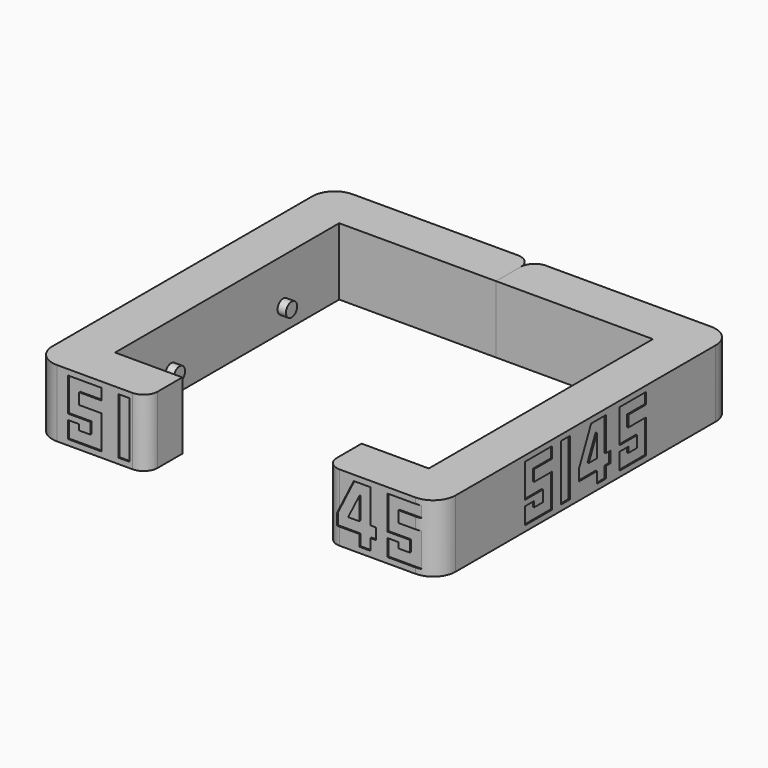
from build123d import *

# Parameters (mm, degrees)
F1_DEPTH       = 15.24
F2_R           = 1.5875
F3_DEPTH       = 1.905
F5_DEPTH       = 15.24
F6_R           = 1.5875
F7_DEPTH       = 1.905
F8_W           = 2.54
F8_H           = 12.7
F9_DEPTH       = 0.79375
F11_DEPTH      = 0.79375
F12_W          = 2.54
F12_H          = 12.7
F13_DEPTH      = 0.79375
F14_W          = 2.54
F14_H          = 12.7
F15_DEPTH      = 0.79375
F16_W          = 2.54
F16_H          = 12.7
F17_DEPTH      = 0.79375
F19_DEPTH      = 0.79375
F20_R          = 5.08
F21_T1_DEPTH   = 40.64
F22_T1_DEPTH   = 31.115
F22_2_T1_DEPTH = 31.115
F23_DEPTH      = 0.5
F24_DEPTH      = 0.5
F25_DEPTH      = 0.5
F26_DEPTH      = 0.5
F27_DEPTH      = 0.5
F28_DEPTH      = 0.5


# Not quite as in the source:
# - a fillet or chamfer that OpenCascade refuses, or shapes differently, is made with other operations: its cross-section is extruded or revolved along the edge and cut away or added


with BuildPart() as f1:
    # F0 (on Top) → F1 (new body)
    with BuildSketch(Plane.XY):
        Polygon((0, 38.8312135783), (0, 28.6712135783), (35.56, 28.6712135783), (35.56, -34.8287864217), (20.32, -34.8287864217), (20.32, -44.9887864217), (45.72, -44.9887864217), (45.72, 38.8312135783), align=None)
    extrude(amount=F1_DEPTH)

    # F2 (on face) → F3 (join)
    with BuildSketch(Plane(origin=(35.56, 0, 0), x_dir=(0, -1, 0), z_dir=(-1, 0, 0))):
        with Locations((-12.7962135783, 5.08)):
            Circle(F2_R)
        with Locations((18.9537864217, 5.08)):
            Circle(F2_R)
    extrude(amount=F3_DEPTH)

    # F8 (on face) → F9 (cut)
    with BuildSketch(Plane.YZ.offset(45.72)):
        Polygon((-12.6037864217, 11.43), (-12.6037864217, 13.97), (-20.2237864217, 13.97), (-20.2237864217, 6.35), (-15.1437864217, 6.35), (-15.1437864217, 3.81), (-17.6837864217, 3.81), (-17.6837864217, 5.08), (-20.2237864217, 5.08), (-20.2237864217, 1.27), (-12.6037864217, 1.27), (-12.6037864217, 8.89), (-17.6837864217, 8.89), (-17.6837864217, 11.43), align=None)
        with Locations((-8.7937864217, 7.62)):
            Rectangle(F8_W, F8_H)
        Polygon((2.6362135783, 13.97), (-1.5439947518, 13.97), (-4.9837864217, 6.35), (-4.9837864217, 3.81), (0.0962135783, 3.81), (0.0962135783, 1.27), (2.6362135783, 1.27), (2.6362135783, 3.81), (3.9062135783, 3.81), (3.9062135783, 6.35), (2.6362135783, 6.35), align=None)
        Polygon((0.0962135783, 11.43), (0.0962135783, 6.35), (-2.1969808683, 6.35), align=None, mode=Mode.SUBTRACT)
        Polygon((14.0662135783, 11.43), (14.0662135783, 13.97), (6.4462135783, 13.97), (6.4462135783, 6.35), (11.5262135783, 6.35), (11.5262135783, 3.81), (8.9862135783, 3.81), (8.9862135783, 5.08), (6.4462135783, 5.08), (6.4462135783, 1.27), (14.0662135783, 1.27), (14.0662135783, 8.89), (8.9862135783, 8.89), (8.9862135783, 11.43), align=None)
    extrude(amount=-F9_DEPTH, mode=Mode.SUBTRACT)

    # F10 (on face) → F11 (cut)
    with BuildSketch(Plane.XZ.offset(44.9887864217)):
        Polygon((26.67, 13.97), (22.86, 6.35), (22.86, 3.81), (27.94, 3.81), (27.94, 1.27), (30.48, 1.27), (30.48, 3.81), (31.75, 3.81), (31.75, 6.35), (30.48, 6.35), (30.48, 13.97), align=None)
        Polygon((27.94, 11.43), (27.94, 6.35), (25.4, 6.35), align=None, mode=Mode.SUBTRACT)
        Polygon((41.91, 11.43), (41.91, 13.97), (34.29, 13.97), (34.29, 6.35), (39.37, 6.35), (39.37, 3.81), (36.83, 3.81), (36.83, 5.08), (34.29, 5.08), (34.29, 1.27), (41.91, 1.27), (41.91, 8.89), (36.83, 8.89), (36.83, 11.43), align=None)
    extrude(amount=-F11_DEPTH, mode=Mode.SUBTRACT)

    # F16 (on face) → F17 (cut)
    with BuildSketch(Plane(origin=(0, 38.8312135783, 0), x_dir=(-1, 0, 0), z_dir=(0, 1, 0))):
        Polygon((-8.89, 11.43), (-8.89, 13.97), (-16.51, 13.97), (-16.51, 6.35), (-11.43, 6.35), (-11.43, 3.81), (-13.97, 3.81), (-13.97, 5.08), (-16.51, 5.08), (-16.51, 1.27), (-8.89, 1.27), (-8.89, 8.89), (-13.97, 8.89), (-13.97, 11.43), align=None)
        with Locations((-5.08, 7.62)):
            Rectangle(F16_W, F16_H)
    extrude(amount=-F17_DEPTH, mode=Mode.SUBTRACT)

    # F21: fillet of radius 5.08 on 2 edges, made by hand

    # F21_s2 → F21_t1 (cut)
    with BuildSketch(Plane.XY.offset(-12.7)):
        with BuildLine():
            ThreePointArc((45.72, -39.9087864217), (44.2321024484, -43.5008888701), (40.64, -44.9887864217))
            Line((40.64, -44.9887864217), (45.72, -44.9887864217))
            Line((45.72, -44.9887864217), (45.72, -39.9087864217))
        make_face()
        with BuildLine():
            ThreePointArc((40.64, 38.8312135783), (44.2321024484, 37.3433160267), (45.72, 33.7512135783))
            Line((45.72, 33.7512135783), (45.72, 38.8312135783))
            Line((45.72, 38.8312135783), (40.64, 38.8312135783))
        make_face()
    extrude(amount=F21_T1_DEPTH, mode=Mode.SUBTRACT)

    # F22: fillet of radius 3.175 on 2 edges, made by hand

    # F22_s2 → F22_t1 (cut)
    with BuildSketch(Plane.XY.offset(-7.9375)):
        with BuildLine():
            ThreePointArc((23.495, -44.9887864217), (21.2499359697, -44.058850452), (20.32, -41.8137864217))
            Line((20.32, -41.8137864217), (20.32, -44.9887864217))
            Line((20.32, -44.9887864217), (23.495, -44.9887864217))
        make_face()
        with BuildLine():
            ThreePointArc((0, 35.6562135783), (0.9299359697, 37.9012776086), (3.175, 38.8312135783))
            Line((3.175, 38.8312135783), (0, 38.8312135783))
            Line((0, 38.8312135783), (0, 35.6562135783))
        make_face()
    extrude(amount=F22_T1_DEPTH, mode=Mode.SUBTRACT)

    # F25 (add): faces of the model
    f25_faces = [f1.faces().sort_by_distance(p)[0] for p in [
        (24.9036570157, -44.1950364217, 10.0906714922),
        (37.9895652174, -44.1950364217, 7.4819565217),
    ]]
    extrude(f25_faces, amount=F25_DEPTH)

    # F26 (add): faces of the model
    f26_faces = [f1.faces().sort_by_distance(p)[0] for p in [
        (44.92625, -16.5242212043, 7.4819565217),
        (44.92625, -8.7937864217, 7.62),
        (44.92625, 3.2712135783, 3.9650232563),
        (44.92625, 10.1457787957, 7.4819565217),
    ]]
    extrude(f26_faces, amount=F26_DEPTH)

    # F27 (add): faces of the model
    f27_faces = [f1.faces().sort_by_distance(p)[0] for p in [
        (12.8104347826, 38.0374635783, 7.4819565217),
        (5.08, 38.0374635783, 7.62),
    ]]
    extrude(f27_faces, amount=F27_DEPTH)


with BuildPart() as f5:
    # F4 (on Top) → F5 (new body)
    with BuildSketch(Plane.XY):
        Polygon((-35.56, 28.6712135783), (0, 28.6712135783), (0, 38.8312135783), (-45.72, 38.8312135783), (-45.72, -44.9887864217), (-20.32, -44.9887864217), (-20.32, -34.8287864217), (-35.56, -34.8287864217), align=None)
    extrude(amount=F5_DEPTH)

    # F6 (on face) → F7 (join)
    with BuildSketch(Plane.YZ.offset(-35.56)):
        with Locations((12.7962135783, 5.08)):
            Circle(F6_R)
        with Locations((-18.9537864217, 5.08)):
            Circle(F6_R)
    extrude(amount=F7_DEPTH)

    # F12 (on face) → F13 (cut)
    with BuildSketch(Plane.XZ.offset(44.9887864217)):
        Polygon((-30.48, 11.43), (-30.48, 13.97), (-38.1, 13.97), (-38.1, 6.35), (-33.02, 6.35), (-33.02, 3.81), (-35.56, 3.81), (-35.56, 5.08), (-38.1, 5.08), (-38.1, 1.27), (-30.48, 1.27), (-30.48, 8.89), (-35.56, 8.89), (-35.56, 11.43), align=None)
        with Locations((-25.4, 7.62)):
            Rectangle(F12_W, F12_H)
    extrude(amount=-F13_DEPTH, mode=Mode.SUBTRACT)

    # F14 (on face) → F15 (cut)
    with BuildSketch(Plane(origin=(-45.72, 0, 0), x_dir=(0, -1, 0), z_dir=(-1, 0, 0))):
        Polygon((-6.4462135783, 11.43), (-6.4462135783, 13.97), (-14.0662135783, 13.97), (-14.0662135783, 6.35), (-8.9862135783, 6.35), (-8.9862135783, 3.81), (-11.5262135783, 3.81), (-11.5262135783, 5.08), (-14.0662135783, 5.08), (-14.0662135783, 1.27), (-6.4462135783, 1.27), (-6.4462135783, 8.89), (-11.5262135783, 8.89), (-11.5262135783, 11.43), align=None)
        with Locations((-2.6362135783, 7.62)):
            Rectangle(F14_W, F14_H)
        Polygon((8.7937864217, 13.97), (4.9837864217, 13.97), (1.1737864217, 6.35), (1.1737864217, 3.81), (6.2537864217, 3.81), (6.2537864217, 1.27), (8.7937864217, 1.27), (8.7937864217, 3.81), (10.0637864217, 3.81), (10.0637864217, 6.35), (8.7937864217, 6.35), align=None)
        Polygon((6.2537864217, 11.43), (6.2537864217, 6.35), (3.7137864217, 6.35), align=None, mode=Mode.SUBTRACT)
        Polygon((20.2237864217, 11.43), (20.2237864217, 13.97), (12.6037864217, 13.97), (12.6037864217, 6.35), (17.6837864217, 6.35), (17.6837864217, 3.81), (15.1437864217, 3.81), (15.1437864217, 5.08), (12.6037864217, 5.08), (12.6037864217, 1.27), (20.2237864217, 1.27), (20.2237864217, 8.89), (15.1437864217, 8.89), (15.1437864217, 11.43), align=None)
    extrude(amount=-F15_DEPTH, mode=Mode.SUBTRACT)

    # F18 (on face) → F19 (cut)
    with BuildSketch(Plane(origin=(0, 38.8312135783, 0), x_dir=(-1, 0, 0), z_dir=(0, 1, 0))):
        Polygon((6.35, 13.97), (2.54, 6.35), (2.54, 3.81), (7.62, 3.81), (7.62, 1.27), (10.16, 1.27), (10.16, 3.81), (11.43, 3.81), (11.43, 6.35), (10.16, 6.35), (10.16, 13.97), align=None)
        Polygon((7.62, 11.43), (7.62, 6.35), (5.08, 6.35), align=None, mode=Mode.SUBTRACT)
        Polygon((21.59, 11.43), (21.59, 13.97), (13.97, 13.97), (13.97, 6.35), (19.05, 6.35), (19.05, 3.81), (16.51, 3.81), (16.51, 5.08), (13.97, 5.08), (13.97, 1.27), (21.59, 1.27), (21.59, 8.89), (16.51, 8.89), (16.51, 11.43), align=None)
    extrude(amount=-F19_DEPTH, mode=Mode.SUBTRACT)

    # F20
    f20_edges = [f5.edges().sort_by_distance(p)[0] for p in [
        (-45.72, 38.831214, 7.62),
        (-45.72, -44.988786, 7.62),
    ]]
    fillet(f20_edges, radius=F20_R)

    # F22#2: fillet of radius 3.175 on 2 edges, made by hand

    # F22_2_s2 → F22_2_t1 (cut)
    with BuildSketch(Plane.XY.offset(-7.9375)):
        with BuildLine():
            ThreePointArc((-23.495, -44.9887864217), (-21.2499359697, -44.058850452), (-20.32, -41.8137864217))
            Line((-20.32, -41.8137864217), (-20.32, -44.9887864217))
            Line((-20.32, -44.9887864217), (-23.495, -44.9887864217))
        make_face()
        with BuildLine():
            ThreePointArc((-3.175, 38.8312135783), (-0.9299359697, 37.9012776086), (0, 35.6562135783))
            Line((0, 35.6562135783), (0, 38.8312135783))
            Line((0, 38.8312135783), (-3.175, 38.8312135783))
        make_face()
    extrude(amount=F22_2_T1_DEPTH, mode=Mode.SUBTRACT)

    # F23 (add): faces of the model
    f23_faces = [f5.faces().sort_by_distance(p)[0] for p in [
        (-44.92625, 10.3666483609, 7.4819565217),
        (-44.92625, 2.6362135783, 7.62),
        (-44.92625, -9.4287864217, 3.9650232563),
        (-44.92625, -16.3033516391, 7.4819565217),
    ]]
    extrude(f23_faces, amount=F23_DEPTH)

    # F24 (add): faces of the model
    f24_faces = [f5.faces().sort_by_distance(p)[0] for p in [
        (-34.4004347826, -44.1950364217, 7.4819565217),
        (-25.4, -44.1950364217, 7.62),
    ]]
    extrude(f24_faces, amount=F24_DEPTH)

    # F28 (add): faces of the model
    f28_faces = [f5.faces().sort_by_distance(p)[0] for p in [
        (-4.5836570157, 38.0374635783, 10.0906714922),
        (-17.6695652174, 38.0374635783, 7.4819565217),
    ]]
    extrude(f28_faces, amount=F28_DEPTH)


solid = Compound([f1.part, f5.part])
